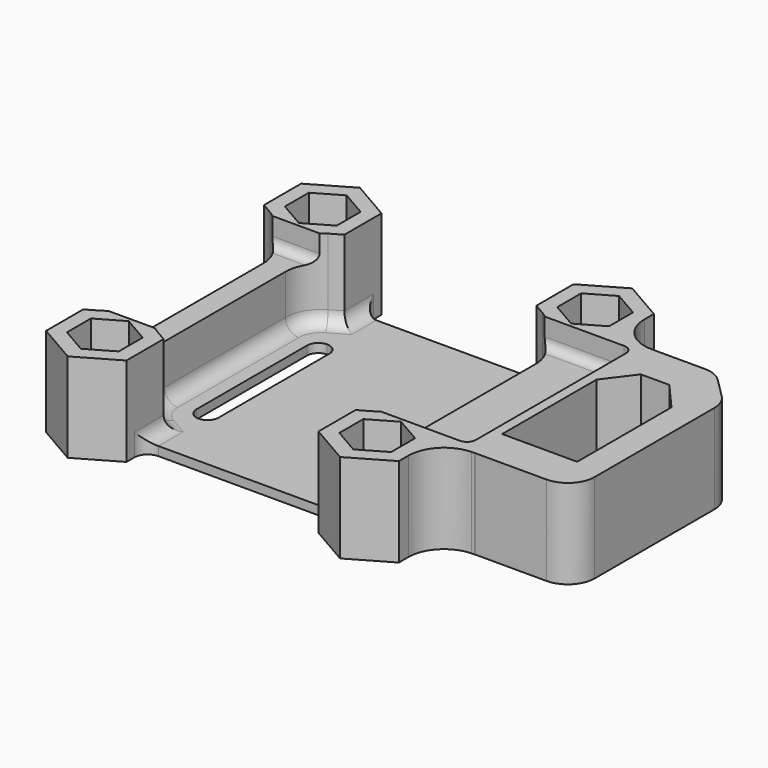
from build123d import *

# Parameters (mm, degrees)
F0_W          = 30.5
F0_H          = 30.5
F1_DEPTH      = 1
F3_DEPTH      = 10
F4_W          = 45
F4_H          = 23
F5_DEPTH      = 3
F7_DEPTH      = 10.001
F8_SIZE       = 4
F9_T1_DEPTH   = 10
F9_T6_DEPTH   = 7
F9_T11_DEPTH  = 7
F9_T16_DEPTH  = 12.7735026919
F9_T23_DEPTH  = 7
F9_T28_DEPTH  = 7
F9_T33_DEPTH  = 12.7735026919
F9_T40_DEPTH  = 6
F9_T45_DEPTH  = 6
F9_T50_DEPTH  = 11.7735026919
F9_T57_DEPTH  = 6
F9_T62_DEPTH  = 6
F9_T67_DEPTH  = 11.7735026919
F9_T74_DEPTH  = 6
F9_T79_DEPTH  = 6
F9_T84_DEPTH  = 11.7735026919
F9_T91_DEPTH  = 6
F9_T96_DEPTH  = 6
F9_T101_DEPTH = 11.7735026919
F10_R         = 1
F11_R         = 1.5
F12_T1_DEPTH  = 2
F12_S5_W      = 1
F12_S5_H      = 1
F12_T6_DEPTH  = 1
F12_S11_W     = 1
F12_S11_H     = 1
F12_T12_DEPTH = 1
F13_R         = 3
F14_R         = 1.5
F16_DEPTH     = 1.0010001


# Not quite as in the source:
# - a fillet or chamfer that OpenCascade refuses, or shapes differently, is made with other operations: its cross-section is extruded or revolved along the edge and cut away or added


with BuildPart() as f1:
    # F0 (on Top) → F1 (new body)
    with BuildSketch(Plane.XY):
        Rectangle(F0_W, F0_H)
    extrude(amount=F1_DEPTH)

    # F2 (on Top) → F3 (join)
    with BuildSketch(Plane.XY):
        Polygon((-19.75, 12.6519237886), (-16.5, 10.7755354138), (-16.5, -10.7755354138), (-19.75, -12.6519237886), (-19.75, -17.8480762114), (-15.25, -20.4461524227), (-10.75, -17.8480762114), (-10.75, -12.6519237886), (-14, -10.7755354138), (-14, 10.7755354138), (-10.75, 12.6519237886), (-10.75, 17.8480762114), (-15.25, 20.4461524227), (-19.75, 17.8480762114), align=None)
        Polygon((24, 12.5), (19.75, 12.6519237886), (19.75, 17.8480762114), (15.25, 20.4461524227), (10.75, 17.8480762114), (10.75, 12.6519237886), (14, 10.7755354138), (14, -10.7755354138), (10.75, -12.6519237886), (10.75, -17.8480762114), (15.25, -20.4461524227), (19.75, -17.8480762114), (19.75, -12.6519237886), (24, -12.5), (35, -12.5), (35, 12.5), align=None)
    extrude(amount=F3_DEPTH)

    # F4 (on face) → F5 (cut)
    with BuildSketch(Plane.XY.offset(10)):
        Rectangle(F4_W, F4_H)
    extrude(amount=-F5_DEPTH, mode=Mode.SUBTRACT)

    # F6 (on face) → F7 (cut, through all)
    with BuildSketch(Plane.XY.offset(10)):
        Polygon((29.2, 8.2), (26, 8.2), (23.6, 5), (23.6, -8.2), (32, -8.2), (32, 5), align=None)
        Polygon((-15.25, 11.9013684387), (-12.35, 13.5756842194), (-12.35, 16.9243157806), (-15.25, 18.5986315613), (-18.15, 16.9243157806), (-18.15, 13.5756842194), align=None)
        Polygon((-12.35, -13.5756842194), (-15.25, -11.9013684387), (-18.15, -13.5756842194), (-18.15, -16.9243157806), (-15.25, -18.5986315613), (-12.35, -16.9243157806), align=None)
        Polygon((15.25, 18.5986315613), (12.35, 16.9243157806), (12.35, 13.5756842194), (15.25, 11.9013684387), (18.15, 13.5756842194), (18.15, 16.9243157806), align=None)
        Polygon((12.35, -13.5756842194), (12.35, -16.9243157806), (15.25, -18.5986315613), (18.15, -16.9243157806), (18.15, -13.5756842194), (15.25, -11.9013684387), align=None)
    extrude(amount=-F7_DEPTH, mode=Mode.SUBTRACT)

    # F8
    f8_edges = [f1.edges().sort_by_distance(p)[0] for p in [
        (35, 12.5, 5),
    ]]
    chamfer(f8_edges, length=F8_SIZE)

    # F9: fillet of radius 4 on 10 edges, made by hand

    # F9_s2 → F9_t1 (join)
    with BuildSketch(Plane.XY):
        with BuildLine():
            ThreePointArc((24.071470723, 12.5), (24.0000114059, 12.5006383552), (23.9285748971, 12.502553217))
            Line((23.9285748971, 12.502553217), (24, 12.5))
            Line((24, 12.5), (24.071470723, 12.5))
        make_face()
        with BuildLine():
            ThreePointArc((23.6071041741, 12.5140447582), (20.8714948929, 13.7340451694), (19.75, 16.5114915412))
            Line((19.75, 16.5114915412), (19.75, 12.6519237886))
            Line((19.75, 12.6519237886), (23.6071041741, 12.5140447582))
        make_face()
        with BuildLine():
            ThreePointArc((23.6071041741, -12.5140447582), (20.8714948929, -13.7340451694), (19.75, -16.5114915412))
            Line((19.75, -16.5114915412), (19.75, -12.6519237886))
            Line((19.75, -12.6519237886), (23.6071041741, -12.5140447582))
        make_face()
        with BuildLine():
            ThreePointArc((24.071470723, -12.5), (24.0000114059, -12.5006383552), (23.9285748971, -12.502553217))
            Line((23.9285748971, -12.502553217), (24, -12.5))
            Line((24, -12.5), (24.071470723, -12.5))
        make_face()
    extrude(amount=F9_T1_DEPTH)


with BuildPart() as f9_tool4:
    # F9_s5 → F9_t6 (new body)
    with BuildSketch(Plane.XY):
        with BuildLine():
            ThreePointArc((-18.5, 11.9302359522), (-17.0358983849, 10.466134337), (-16.5, 8.466134337))
            Line((-16.5, 8.466134337), (-16.5, 10.7755354138))
            Line((-16.5, 10.7755354138), (-18.5, 11.9302359522))
        make_face()
    extrude(amount=F9_T6_DEPTH)

    split(bisect_by=Plane.XZ.offset(-11.5), keep=Keep.BOTTOM)


with BuildPart() as f1_1:
    add(f1.part)

    # F9_t3: union F9_tool4
    add(f9_tool4.part)


with BuildPart() as f9_tool9:
    # F9_s10 → F9_t11 (new body)
    with BuildSketch(Plane.XY):
        with BuildLine():
            ThreePointArc((-18.5, 11.9302359522), (-17.0358983849, 10.466134337), (-16.5, 8.466134337))
            Line((-16.5, 8.466134337), (-16.5, 10.7755354138))
            Line((-16.5, 10.7755354138), (-18.5, 11.9302359522))
        make_face()
    extrude(amount=F9_T11_DEPTH)

    split(bisect_by=Plane.XZ.offset(-11.5), keep=Keep.TOP)


with BuildPart() as f1_2:
    add(f1_1.part)

    # F9_t8: union F9_tool9
    add(f9_tool9.part)


with BuildPart() as f9_tool14:
    # F9_s15 → F9_t16 (new body)
    with BuildSketch(Plane.XY):
        with BuildLine():
            ThreePointArc((-18.5, 11.9302359522), (-17.0358983849, 10.466134337), (-16.5, 8.466134337))
            Line((-16.5, 8.466134337), (-16.5, 10.7755354138))
            Line((-16.5, 10.7755354138), (-18.5, 11.9302359522))
        make_face()
    extrude(amount=F9_T16_DEPTH)

    split(bisect_by=Plane.XY.offset(7), keep=Keep.TOP)

    split(bisect_by=Plane.XZ.offset(-11.5), keep=Keep.BOTTOM)

    split(bisect_by=Plane.XY.offset(10), keep=Keep.BOTTOM)


with BuildPart() as f1_3:
    add(f1_2.part)

    # F9_t13: union F9_tool14
    add(f9_tool14.part)


with BuildPart() as f9_tool21:
    # F9_s22 → F9_t23 (new body)
    with BuildSketch(Plane.XY):
        with BuildLine():
            ThreePointArc((-18.5, -11.9302359522), (-17.0358983849, -10.466134337), (-16.5, -8.466134337))
            Line((-16.5, -8.466134337), (-16.5, -10.7755354138))
            Line((-16.5, -10.7755354138), (-18.5, -11.9302359522))
        make_face()
    extrude(amount=F9_T23_DEPTH)

    split(bisect_by=Plane.XZ.offset(11.5), keep=Keep.TOP)


with BuildPart() as f1_4:
    add(f1_3.part)

    # F9_t20: union F9_tool21
    add(f9_tool21.part)


with BuildPart() as f9_tool26:
    # F9_s27 → F9_t28 (new body)
    with BuildSketch(Plane.XY):
        with BuildLine():
            ThreePointArc((-18.5, -11.9302359522), (-17.0358983849, -10.466134337), (-16.5, -8.466134337))
            Line((-16.5, -8.466134337), (-16.5, -10.7755354138))
            Line((-16.5, -10.7755354138), (-18.5, -11.9302359522))
        make_face()
    extrude(amount=F9_T28_DEPTH)

    split(bisect_by=Plane.XZ.offset(11.5), keep=Keep.BOTTOM)


with BuildPart() as f1_5:
    add(f1_4.part)

    # F9_t25: union F9_tool26
    add(f9_tool26.part)


with BuildPart() as f9_tool31:
    # F9_s32 → F9_t33 (new body)
    with BuildSketch(Plane.XY):
        with BuildLine():
            ThreePointArc((-18.5, -11.9302359522), (-17.0358983849, -10.466134337), (-16.5, -8.466134337))
            Line((-16.5, -8.466134337), (-16.5, -10.7755354138))
            Line((-16.5, -10.7755354138), (-18.5, -11.9302359522))
        make_face()
    extrude(amount=F9_T33_DEPTH)

    split(bisect_by=Plane.XY.offset(10), keep=Keep.BOTTOM)

    split(bisect_by=Plane.XZ.offset(11.5), keep=Keep.TOP)

    split(bisect_by=Plane.XY.offset(7), keep=Keep.TOP)


with BuildPart() as f1_6:
    add(f1_5.part)

    # F9_t30: union F9_tool31
    add(f9_tool31.part)


with BuildPart() as f9_tool38:
    # F9_s39 → F9_t40 (new body)
    with BuildSketch(Plane.XY.offset(1)):
        with BuildLine():
            ThreePointArc((-12, 11.9302359522), (-13.4641016151, 10.466134337), (-14, 8.466134337))
            Line((-14, 8.466134337), (-14, 10.7755354138))
            Line((-14, 10.7755354138), (-12, 11.9302359522))
        make_face()
    extrude(amount=F9_T40_DEPTH)

    split(bisect_by=Plane.XZ.offset(-11.5), keep=Keep.BOTTOM)


with BuildPart() as f1_7:
    add(f1_6.part)

    # F9_t37: union F9_tool38
    add(f9_tool38.part)


with BuildPart() as f9_tool43:
    # F9_s44 → F9_t45 (new body)
    with BuildSketch(Plane.XY.offset(1)):
        with BuildLine():
            ThreePointArc((-12, 11.9302359522), (-13.4641016151, 10.466134337), (-14, 8.466134337))
            Line((-14, 8.466134337), (-14, 10.7755354138))
            Line((-14, 10.7755354138), (-12, 11.9302359522))
        make_face()
    extrude(amount=F9_T45_DEPTH)

    split(bisect_by=Plane.XZ.offset(-11.5), keep=Keep.TOP)


with BuildPart() as f1_8:
    add(f1_7.part)

    # F9_t42: union F9_tool43
    add(f9_tool43.part)


with BuildPart() as f9_tool48:
    # F9_s49 → F9_t50 (new body)
    with BuildSketch(Plane.XY.offset(1)):
        with BuildLine():
            ThreePointArc((-12, 11.9302359522), (-13.4641016151, 10.466134337), (-14, 8.466134337))
            Line((-14, 8.466134337), (-14, 10.7755354138))
            Line((-14, 10.7755354138), (-12, 11.9302359522))
        make_face()
    extrude(amount=F9_T50_DEPTH)

    split(bisect_by=Plane.XY.offset(10), keep=Keep.BOTTOM)

    split(bisect_by=Plane.XZ.offset(-11.5), keep=Keep.BOTTOM)

    split(bisect_by=Plane.XY.offset(7), keep=Keep.TOP)


with BuildPart() as f1_9:
    add(f1_8.part)

    # F9_t47: union F9_tool48
    add(f9_tool48.part)


with BuildPart() as f9_tool55:
    # F9_s56 → F9_t57 (new body)
    with BuildSketch(Plane.XY.offset(1)):
        with BuildLine():
            ThreePointArc((-12, -11.9302359522), (-13.4641016151, -10.466134337), (-14, -8.466134337))
            Line((-14, -8.466134337), (-14, -10.7755354138))
            Line((-14, -10.7755354138), (-12, -11.9302359522))
        make_face()
    extrude(amount=F9_T57_DEPTH)

    split(bisect_by=Plane.XZ.offset(11.5), keep=Keep.TOP)


with BuildPart() as f1_10:
    add(f1_9.part)

    # F9_t54: union F9_tool55
    add(f9_tool55.part)


with BuildPart() as f9_tool60:
    # F9_s61 → F9_t62 (new body)
    with BuildSketch(Plane.XY.offset(1)):
        with BuildLine():
            ThreePointArc((-12, -11.9302359522), (-13.4641016151, -10.466134337), (-14, -8.466134337))
            Line((-14, -8.466134337), (-14, -10.7755354138))
            Line((-14, -10.7755354138), (-12, -11.9302359522))
        make_face()
    extrude(amount=F9_T62_DEPTH)

    split(bisect_by=Plane.XZ.offset(11.5), keep=Keep.BOTTOM)


with BuildPart() as f1_11:
    add(f1_10.part)

    # F9_t59: union F9_tool60
    add(f9_tool60.part)


with BuildPart() as f9_tool65:
    # F9_s66 → F9_t67 (new body)
    with BuildSketch(Plane.XY.offset(1)):
        with BuildLine():
            ThreePointArc((-12, -11.9302359522), (-13.4641016151, -10.466134337), (-14, -8.466134337))
            Line((-14, -8.466134337), (-14, -10.7755354138))
            Line((-14, -10.7755354138), (-12, -11.9302359522))
        make_face()
    extrude(amount=F9_T67_DEPTH)

    split(bisect_by=Plane.XY.offset(7), keep=Keep.TOP)

    split(bisect_by=Plane.XZ.offset(11.5), keep=Keep.TOP)

    split(bisect_by=Plane.XY.offset(10), keep=Keep.BOTTOM)


with BuildPart() as f1_12:
    add(f1_11.part)

    # F9_t64: union F9_tool65
    add(f9_tool65.part)


with BuildPart() as f9_tool72:
    # F9_s73 → F9_t74 (new body)
    with BuildSketch(Plane.XY.offset(1)):
        with BuildLine():
            ThreePointArc((12, 11.9302359522), (13.4641016151, 10.466134337), (14, 8.466134337))
            Line((14, 8.466134337), (14, 10.7755354138))
            Line((14, 10.7755354138), (12, 11.9302359522))
        make_face()
    extrude(amount=F9_T74_DEPTH)

    split(bisect_by=Plane.XZ.offset(-11.5), keep=Keep.BOTTOM)


with BuildPart() as f1_13:
    add(f1_12.part)

    # F9_t71: union F9_tool72
    add(f9_tool72.part)


with BuildPart() as f9_tool77:
    # F9_s78 → F9_t79 (new body)
    with BuildSketch(Plane.XY.offset(1)):
        with BuildLine():
            ThreePointArc((12, 11.9302359522), (13.4641016151, 10.466134337), (14, 8.466134337))
            Line((14, 8.466134337), (14, 10.7755354138))
            Line((14, 10.7755354138), (12, 11.9302359522))
        make_face()
    extrude(amount=F9_T79_DEPTH)

    split(bisect_by=Plane.XZ.offset(-11.5), keep=Keep.TOP)


with BuildPart() as f1_14:
    add(f1_13.part)

    # F9_t76: union F9_tool77
    add(f9_tool77.part)


with BuildPart() as f9_tool82:
    # F9_s83 → F9_t84 (new body)
    with BuildSketch(Plane.XY.offset(1)):
        with BuildLine():
            ThreePointArc((12, 11.9302359522), (13.4641016151, 10.466134337), (14, 8.466134337))
            Line((14, 8.466134337), (14, 10.7755354138))
            Line((14, 10.7755354138), (12, 11.9302359522))
        make_face()
    extrude(amount=F9_T84_DEPTH)

    split(bisect_by=Plane.XY.offset(10), keep=Keep.BOTTOM)

    split(bisect_by=Plane.XY.offset(7), keep=Keep.TOP)

    split(bisect_by=Plane.XZ.offset(-11.5), keep=Keep.BOTTOM)


with BuildPart() as f1_15:
    add(f1_14.part)

    # F9_t81: union F9_tool82
    add(f9_tool82.part)


with BuildPart() as f9_tool89:
    # F9_s90 → F9_t91 (new body)
    with BuildSketch(Plane.XY.offset(1)):
        with BuildLine():
            ThreePointArc((12, -11.9302359522), (13.4641016151, -10.466134337), (14, -8.466134337))
            Line((14, -8.466134337), (14, -10.7755354138))
            Line((14, -10.7755354138), (12, -11.9302359522))
        make_face()
    extrude(amount=F9_T91_DEPTH)

    split(bisect_by=Plane.XZ.offset(11.5), keep=Keep.TOP)


with BuildPart() as f1_16:
    add(f1_15.part)

    # F9_t88: union F9_tool89
    add(f9_tool89.part)


with BuildPart() as f9_tool94:
    # F9_s95 → F9_t96 (new body)
    with BuildSketch(Plane.XY.offset(1)):
        with BuildLine():
            ThreePointArc((12, -11.9302359522), (13.4641016151, -10.466134337), (14, -8.466134337))
            Line((14, -8.466134337), (14, -10.7755354138))
            Line((14, -10.7755354138), (12, -11.9302359522))
        make_face()
    extrude(amount=F9_T96_DEPTH)

    split(bisect_by=Plane.XZ.offset(11.5), keep=Keep.BOTTOM)


with BuildPart() as f1_17:
    add(f1_16.part)

    # F9_t93: union F9_tool94
    add(f9_tool94.part)


with BuildPart() as f9_tool99:
    # F9_s100 → F9_t101 (new body)
    with BuildSketch(Plane.XY.offset(1)):
        with BuildLine():
            ThreePointArc((12, -11.9302359522), (13.4641016151, -10.466134337), (14, -8.466134337))
            Line((14, -8.466134337), (14, -10.7755354138))
            Line((14, -10.7755354138), (12, -11.9302359522))
        make_face()
    extrude(amount=F9_T101_DEPTH)

    split(bisect_by=Plane.XY.offset(10), keep=Keep.BOTTOM)

    split(bisect_by=Plane.XZ.offset(11.5), keep=Keep.TOP)

    split(bisect_by=Plane.XY.offset(7), keep=Keep.TOP)


with BuildPart() as f1_18:
    add(f1_17.part)

    # F9_t98: union F9_tool99
    add(f9_tool99.part)

    # F10
    f10_edges = [f1_18.edges().sort_by_distance(p)[0] for p in [
        (-15.25, -11.5, 7),
        (-15.25, 11.5, 7),
        (17.553424, 11.5, 7),
        (17.553424, -11.5, 7),
        (22.5, 0, 7),
    ]]
    fillet(f10_edges, radius=F10_R)

    # F11
    f11_edges = [f1_18.edges().sort_by_distance(p)[0] for p in [
        (-13.464102, -10.466134, 1),
        (-10.75, -13.950962, 1),
        (-10.75, 13.950962, 1),
        (14, 0, 1),
        (10.75, 13.950962, 1),
        (10.75, -13.950962, 1),
    ]]
    fillet(f11_edges, radius=F11_R)

    # F12: fillet of radius 1 on 2 edges, made by hand

    # F12_s2 → F12_t1 (join)
    with BuildSketch(Plane.XY.offset(8)):
        with BuildLine():
            ThreePointArc((21.5, 11.5), (22.2071067812, 11.2071067812), (22.5, 10.5))
            Line((22.5, 10.5), (22.5, 11.5))
            Line((22.5, 11.5), (21.5, 11.5))
        make_face()
        with BuildLine():
            ThreePointArc((21.5, -11.5), (22.2071067812, -11.2071067812), (22.5, -10.5))
            Line((22.5, -10.5), (22.5, -11.5))
            Line((22.5, -11.5), (21.5, -11.5))
        make_face()
    extrude(amount=F12_T1_DEPTH)


with BuildPart() as f12_tool4:
    # F12_s5 → F12_t6 (new body)
    with BuildSketch(Plane.XZ.offset(10.5)):
        with Locations((22, 7.5)):
            Rectangle(F12_S5_W, F12_S5_H)
    extrude(amount=F12_T6_DEPTH)

    # F12_s7 → F12_t8 (revolve, cut)
    with BuildSketch(Plane(origin=(21.5, -10.5, 8), x_dir=(-0.7071067812, 0, 0.7071067812), z_dir=(0.7071067812, 0, 0.7071067812))):
        with BuildLine():
            ThreePointArc((0, -1), (1, 0), (0, 1))
            Line((0, 1), (0, -1))
        make_face()
    revolve(axis=Axis((21.5, -10.5, 8), (0, -1, 0)), mode=Mode.SUBTRACT)


with BuildPart() as f1_19:
    add(f1_18.part)

    # F12_t3: union F12_tool4
    add(f12_tool4.part)


with BuildPart() as f12_tool10:
    # F12_s11 → F12_t12 (new body)
    with BuildSketch(Plane.XZ.offset(-10.5)):
        with Locations((22, 7.5)):
            Rectangle(F12_S11_W, F12_S11_H)
    extrude(amount=-F12_T12_DEPTH)

    # F12_s13 → F12_t14 (revolve, cut)
    with BuildSketch(Plane(origin=(21.5, 10.5, 8), x_dir=(-0.7071067812, 0, 0.7071067812), z_dir=(-0.7071067812, 0, -0.7071067812))):
        with BuildLine():
            ThreePointArc((0, -1), (1, 0), (0, 1))
            Line((0, 1), (0, -1))
        make_face()
    revolve(axis=Axis((21.5, 10.5, 8), (0, 1, 0)), mode=Mode.SUBTRACT)


with BuildPart() as f1_20:
    add(f1_19.part)

    # F12_t9: union F12_tool10
    add(f12_tool10.part)

    # F13
    f13_edges = [f1_20.edges().sort_by_distance(p)[0] for p in [
        (35, -12.5, 5),
        (35, 8.5, 5),
        (31, 12.5, 5),
    ]]
    fillet(f13_edges, radius=F13_R)

    # F14
    f14_edges = [f1_20.edges().sort_by_distance(p)[0] for p in [
        (10.75, 15.25, 1.25),
        (-10.75, 15.25, 1.25),
        (-10.75, -15.25, 1.25),
        (10.75, -15.25, 1.25),
    ]]
    fillet(f14_edges, radius=F14_R)

    # F15 (on face) → F16 (cut, through all)
    with BuildSketch(Plane.XY.offset(1)):
        with BuildLine():
            ThreePointArc((-9.75, 9), (-10.6338834765, 8.6338834765), (-11, 7.75))
            Line((-11, 7.75), (-11, -7.75))
            ThreePointArc((-11, -7.75), (-10.6338834765, -8.6338834765), (-9.75, -9))
            ThreePointArc((-9.75, -9), (-8.8661165235, -8.6338834765), (-8.5, -7.75))
            Line((-8.5, -7.75), (-8.5, 7.75))
            ThreePointArc((-8.5, 7.75), (-8.8661165235, 8.6338834765), (-9.75, 9))
        make_face()
        with BuildLine():
            ThreePointArc((8.5, -7.75), (8.8661165235, -8.6338834765), (9.75, -9))
            ThreePointArc((9.75, -9), (10.6338834765, -8.6338834765), (11, -7.75))
            Line((11, -7.75), (11, 7.75))
            ThreePointArc((11, 7.75), (10.6338834765, 8.6338834765), (9.75, 9))
            ThreePointArc((9.75, 9), (8.8661165235, 8.6338834765), (8.5, 7.75))
            Line((8.5, 7.75), (8.5, -7.75))
        make_face()
    extrude(amount=-F16_DEPTH, mode=Mode.SUBTRACT)


solid = f1_20.part
